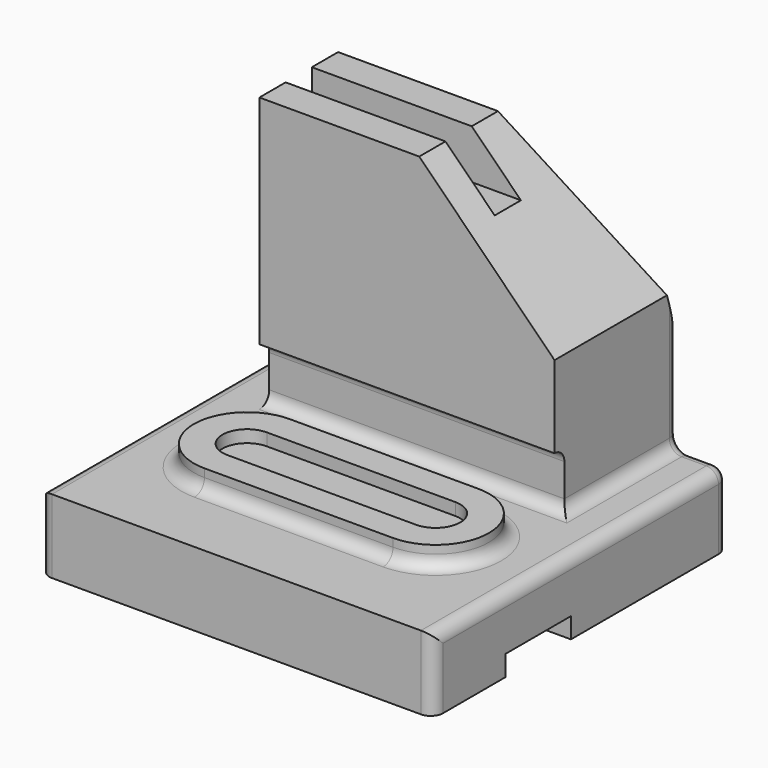
from build123d import *

# Parameters (mm, degrees)
F0_W      = 96
F0_H      = 90
F1_DEPTH  = 18
F2_W      = 72
F2_H      = 38
F4_DEPTH  = 67
F6_DEPTH  = 38
F7_W      = 8
F7_H      = 12
F8_DEPTH  = 51.001
F10_DEPTH = 72.001
F11_W     = 20
F11_H     = 5
F12_DEPTH = 96
F13_W     = 46
F13_H     = 26
F14_DEPTH = 5
F16_DEPTH = 3
F17_W     = 3
F17_H     = 14
F18_DEPTH = 72
F19_R     = 2.99999


# Not quite as in the source:
# - a fillet or chamfer is up to 0.001 mm smaller than in the source, because OpenCascade refuses the exact size


with BuildPart() as f1:
    # F0 (on Top) → F1 (new body)
    with BuildSketch(Plane.XY):
        with Locations((48, 45)):
            Rectangle(F0_W, F0_H)
    extrude(amount=F1_DEPTH)

    # F2 (on face) → F4 (join, through all)
    with BuildSketch(Plane.XY.offset(18)):
        with Locations((48, 71)):
            Rectangle(F2_W, F2_H)
    extrude(amount=F4_DEPTH)

    # F5 (on face) → F6 (cut)
    with BuildSketch(Plane.XZ.offset(-52)):
        Polygon((84, 52), (84, 85), (51, 85), align=None)
    extrude(amount=-F6_DEPTH, mode=Mode.SUBTRACT)

    # F7 (on face) → F8 (cut, through all)
    with BuildSketch(Plane(origin=(12, 0, 0), x_dir=(0, -1, 0), z_dir=(-1, 0, 0))):
        with Locations((-64, 79)):
            Rectangle(F7_W, F7_H)
    extrude(amount=-F8_DEPTH, mode=Mode.SUBTRACT)

    # F9 (on face) → F10 (cut, through all)
    with BuildSketch(Plane(origin=(12, 0, 0), x_dir=(0, -1, 0), z_dir=(-1, 0, 0))):
        Polygon((-76, 85), (-90, 85), (-90, 40), align=None)
    extrude(amount=-F10_DEPTH, mode=Mode.SUBTRACT)

    # F11 (on face) → F12 (cut, through all)
    with BuildSketch(Plane.YZ.offset(96)):
        with Locations((32, 2.5)):
            Rectangle(F11_W, F11_H)
    extrude(amount=-F12_DEPTH, mode=Mode.SUBTRACT)

    # F13 (on face) → F14 (join)
    with BuildSketch(Plane.XY.offset(18)):
        with Locations((48, 32)):
            Rectangle(F13_W, F13_H)
        with BuildLine():
            Line((25, 19), (25, 45))
            ThreePointArc((25, 45), (12, 32), (25, 19))
        make_face()
        with BuildLine():
            ThreePointArc((71, 19), (84, 32), (71, 45))
            Line((71, 45), (71, 19))
        make_face()
    extrude(amount=F14_DEPTH)

    # F15 (on face) → F16 (cut)
    with BuildSketch(Plane.XY.offset(23)):
        with BuildLine():
            ThreePointArc((25, 38), (19, 32), (25, 26))
            Line((25, 26), (71, 26))
            ThreePointArc((71, 26), (77, 32), (71, 38))
            Line((71, 38), (25, 38))
        make_face()
    extrude(amount=-F16_DEPTH, mode=Mode.SUBTRACT)

    # F17 (on face) → F18 (cut, through all)
    with BuildSketch(Plane.YZ.offset(84)):
        with Locations((53.5, 25)):
            Rectangle(F17_W, F17_H)
    extrude(amount=-F18_DEPTH, mode=Mode.SUBTRACT)

    # F19 (radius 3 in the source; OpenCascade refuses exactly that, so slightly less here)
    f19_edges = [f1.edges().sort_by_distance(p)[0] for p in [
        (48, 19, 18),
        (48, 55, 18),
        (48, 55, 32),
        (90, 90, 18),
        (96, 0, 9),
        (96, 90, 9),
        (0, 90, 9),
        (0, 0, 9),
        (0, 45, 18),
        (96, 45, 18),
        (84, 72.5, 18),
        (48, 45, 18),
        (84, 32, 18),
        (12, 32, 18),
        (84, 90, 29),
    ]]
    fillet(f19_edges, radius=F19_R)


solid = f1.part
